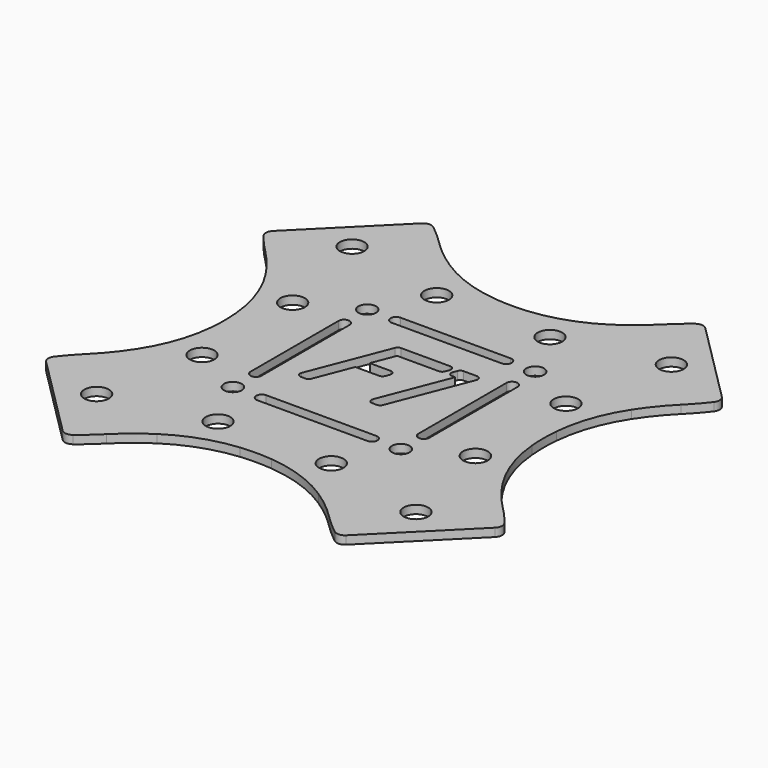
from build123d import *

# Parameters (mm, degrees)
F0_R     = 2.225
F0_R_2   = 1.6
F0_R_3   = 2.25
F1_DEPTH = 1.5


# Not quite as in the source:
# - ends of sketch curves that miss each other by under 0.0002 mm in the source are joined


with BuildPart() as f1:
    # F0 (on Top) → F1 (new body)
    with BuildSketch(Plane.XY):
        with BuildLine():
            Line((40.764131, 25.752812), (25.752812, 40.764131))
            ThreePointArc((25.752812, 40.764131), (24.7844707903, 41.2006273849), (23.7698381424, 40.8864068174))
            ThreePointArc((23.7698381424, 40.8864068174), (21.9550704325, 39.3793732762), (20.2364945752, 37.7635054248))
            ThreePointArc((20.2364945752, 37.7635054248), (17.5612326137, 35.3520830837), (14.6508446305, 33.2303795663))
            ThreePointArc((14.6508446305, 33.2303795663), (8.9914965544, 30.4470141229), (2.8299590067, 29.1013549294))
            ThreePointArc((2.8299590067, 29.1013549294), (0, 28.968262), (-2.8299590155, 29.1013548358))
            ThreePointArc((-2.8299590155, 29.1013548358), (-8.9914965544, 30.4470141229), (-14.6508445509, 33.2303796882))
            ThreePointArc((-14.6508445509, 33.2303796882), (-17.5612326137, 35.3520830837), (-20.2364941171, 37.7635058829))
            ThreePointArc((-20.2364941171, 37.7635058829), (-21.9550704325, 39.3793732762), (-23.7698383319, 40.8864065743))
            ThreePointArc((-23.7698383319, 40.8864065743), (-24.7844707903, 41.2006273849), (-25.7528121718, 40.7641311718))
            Line((-25.7528121718, 40.7641311718), (-40.764131, 25.752812))
            ThreePointArc((-40.764131, 25.752812), (-41.2006273849, 24.7844707903), (-40.8864068174, 23.7698381424))
            ThreePointArc((-40.8864068174, 23.7698381424), (-39.3793732762, 21.9550704325), (-37.7635054248, 20.2364945752))
            ThreePointArc((-37.7635054248, 20.2364945752), (-35.3520832558, 17.5612328258), (-33.2303798649, 14.6508450882))
            ThreePointArc((-33.2303798649, 14.6508450882), (-30.4470115556, 8.9914892045), (-29.1013534168, 2.8299429607))
            ThreePointArc((-29.1013534168, 2.8299429607), (-28.968262, 0), (-29.1013532045, -2.8299429807))
            ThreePointArc((-29.1013532045, -2.8299429807), (-30.4470115556, -8.9914892045), (-33.2303799868, -14.6508450086))
            ThreePointArc((-33.2303799868, -14.6508450086), (-35.3520832558, -17.5612328258), (-37.7635058829, -20.2364941171))
            ThreePointArc((-37.7635058829, -20.2364941171), (-39.3793732762, -21.9550704325), (-40.8864065743, -23.7698383319))
            ThreePointArc((-40.8864065743, -23.7698383319), (-41.2006273849, -24.7844707903), (-40.7641311718, -25.7528121718))
            Line((-40.7641311718, -25.7528121718), (-25.752812, -40.764131))
            ThreePointArc((-25.752812, -40.764131), (-24.7844707903, -41.2006273849), (-23.7698381424, -40.8864068174))
            ThreePointArc((-23.7698381424, -40.8864068174), (-21.9550704325, -39.3793732762), (-20.2364945752, -37.7635054248))
            ThreePointArc((-20.2364945752, -37.7635054248), (-17.5612326137, -35.3520830837), (-14.6508446305, -33.2303795663))
            ThreePointArc((-14.6508446305, -33.2303795663), (-8.9914965544, -30.4470141229), (-2.8299590067, -29.1013549294))
            ThreePointArc((-2.8299590067, -29.1013549294), (0, -28.968262), (2.8299590155, -29.1013548358))
            ThreePointArc((2.8299590155, -29.1013548358), (8.9914965544, -30.4470141229), (14.6508445509, -33.2303796882))
            ThreePointArc((14.6508445509, -33.2303796882), (17.5612326137, -35.3520830837), (20.2364941171, -37.7635058829))
            ThreePointArc((20.2364941171, -37.7635058829), (21.9550704325, -39.3793732762), (23.7698383319, -40.8864065743))
            ThreePointArc((23.7698383319, -40.8864065743), (24.7844707903, -41.2006273849), (25.7528121718, -40.7641311718))
            Line((25.7528121718, -40.7641311718), (40.764131, -25.752812))
            ThreePointArc((40.764131, -25.752812), (41.2006273849, -24.7844707903), (40.8864068174, -23.7698381424))
            ThreePointArc((40.8864068174, -23.7698381424), (39.3793732762, -21.9550704325), (37.7635054248, -20.2364945752))
            ThreePointArc((37.7635054248, -20.2364945752), (35.3520832558, -17.5612328258), (33.2303798649, -14.6508450882))
            ThreePointArc((33.2303798649, -14.6508450882), (30.4470115556, -8.9914892045), (29.1013534168, -2.8299429607))
            ThreePointArc((29.1013534168, -2.8299429607), (28.968262, 0), (29.1013532045, 2.8299429807))
            ThreePointArc((29.1013532045, 2.8299429807), (30.4470115556, 8.9914892045), (33.2303799868, 14.6508450086))
            ThreePointArc((33.2303799868, 14.6508450086), (35.3520832558, 17.5612328258), (37.7635058829, 20.2364941171))
            ThreePointArc((37.7635058829, 20.2364941171), (39.3793732762, 21.9550704325), (40.8864065743, 23.7698383319))
            ThreePointArc((40.8864065743, 23.7698383319), (41.2006273849, 24.7844707903), (40.764131, 25.752812))
        make_face()
        with Locations((-29, -29)):
            Circle(F0_R, mode=Mode.SUBTRACT)
        with Locations((-10.282726, -24.824696)):
            Circle(F0_R, mode=Mode.SUBTRACT)
        with Locations((-24.824696, -10.282726)):
            Circle(F0_R, mode=Mode.SUBTRACT)
        with Locations((-15.25, -15.25)):
            Circle(F0_R_2, mode=Mode.SUBTRACT)
        with Locations((10.282726, -24.824696)):
            Circle(F0_R, mode=Mode.SUBTRACT)
        with Locations((29, -29)):
            Circle(F0_R, mode=Mode.SUBTRACT)
        with BuildLine():
            Line((-10, -14.25), (10, -14.25))
            ThreePointArc((10, -14.25), (11, -15.25), (10, -16.25))
            Line((10, -16.25), (-10, -16.25))
            ThreePointArc((-10, -16.25), (-11, -15.25), (-10, -14.25))
        make_face(mode=Mode.SUBTRACT)
        with Locations((15.25, -15.25)):
            Circle(F0_R_2, mode=Mode.SUBTRACT)
        with Locations((24.824696, -10.282726)):
            Circle(F0_R_3, mode=Mode.SUBTRACT)
        with Locations((-24.824696, 10.282726)):
            Circle(F0_R, mode=Mode.SUBTRACT)
        with BuildLine():
            ThreePointArc((-16.25, 10), (-15.25, 11), (-14.25, 10))
            Line((-14.25, 10), (-14.25, -10))
            ThreePointArc((-14.25, -10), (-15.25, -11), (-16.25, -10))
            Line((-16.25, -10), (-16.25, 10))
        make_face(mode=Mode.SUBTRACT)
        with BuildLine():
            ThreePointArc((-0.4956958589, 0.885209945), (-0.771266673, 0.5382796173), (-1.194556, 0.407413))
            Line((-1.194556, 0.407413), (-5.541795, 0.407413))
            Line((-5.541795, 0.407413), (-8.150595, -6.290485))
            ThreePointArc((-8.150595, -6.290485), (-8.426165673, -6.6374153827), (-8.849455, -6.768282))
            Line((-8.849455, -6.768282), (-9.669691, -6.768282))
            ThreePointArc((-9.669691, -6.768282), (-10.2888243827, -6.441571327), (-10.3685511411, -5.746078945))
            Line((-10.3685511411, -5.746078945), (-4.809405, 8.526614))
            ThreePointArc((-4.809405, 8.526614), (-4.533834327, 8.8735443827), (-4.110545, 9.004411))
            Line((-4.110545, 9.004411), (4.809691, 9.004411))
            ThreePointArc((4.809691, 9.004411), (5.4288241198, 8.6777007117), (5.5085514793, 7.9822088133))
            Line((5.5085514793, 7.9822088133), (5.23237, 7.273132))
            ThreePointArc((5.23237, 7.273132), (4.9567984768, 6.9262017197), (4.533509, 6.795335))
            Line((4.533509, 6.795335), (-3.05373, 6.795335))
            Line((-3.05373, 6.795335), (-4.681371, 2.61649))
            Line((-4.681371, 2.61649), (-0.918374, 2.61649))
            ThreePointArc((-0.918374, 2.61649), (-0.2992406173, 2.289779327), (-0.2195138589, 1.594286945))
            Line((-0.2195138589, 1.594286945), (-0.4956958589, 0.885209945))
        make_face(mode=Mode.SUBTRACT)
        with Locations((-15.25, 15.25)):
            Circle(F0_R_2, mode=Mode.SUBTRACT)
        with Locations((-29, 29)):
            Circle(F0_R, mode=Mode.SUBTRACT)
        with Locations((-10.282726, 24.824696)):
            Circle(F0_R, mode=Mode.SUBTRACT)
        with BuildLine():
            ThreePointArc((3.290309, -6.768282), (2.6711756173, -6.441571327), (2.5914488589, -5.746078945))
            Line((2.5914488589, -5.746078945), (7.47627, 6.795335))
            Line((7.47627, 6.795335), (6.953273, 6.795335))
            ThreePointArc((6.953273, 6.795335), (6.3341396173, 7.122045673), (6.2544128589, 7.817538055))
            Line((6.2544128589, 7.817538055), (6.530595, 8.526614))
            ThreePointArc((6.530595, 8.526614), (6.806165673, 8.8735443827), (7.229455, 9.004411))
            Line((7.229455, 9.004411), (9.669691, 9.004411))
            ThreePointArc((9.669691, 9.004411), (10.2888241198, 8.6777007117), (10.3685514793, 7.9822088133))
            Line((10.3685514793, 7.9822088133), (4.809405, -6.290485))
            ThreePointArc((4.809405, -6.290485), (4.533834327, -6.6374153827), (4.110545, -6.768282))
            Line((4.110545, -6.768282), (3.290309, -6.768282))
        make_face(mode=Mode.SUBTRACT)
        with BuildLine():
            Line((14.25, -10), (14.25, 10))
            ThreePointArc((14.25, 10), (15.25, 11), (16.25, 10))
            Line((16.25, 10), (16.25, -10))
            ThreePointArc((16.25, -10), (15.25, -11), (14.25, -10))
        make_face(mode=Mode.SUBTRACT)
        with BuildLine():
            ThreePointArc((10, 16.25), (11, 15.25), (10, 14.25))
            Line((10, 14.25), (-10, 14.25))
            ThreePointArc((-10, 14.25), (-11, 15.25), (-10, 16.25))
            Line((-10, 16.25), (10, 16.25))
        make_face(mode=Mode.SUBTRACT)
        with Locations((15.25, 15.25)):
            Circle(F0_R_2, mode=Mode.SUBTRACT)
        with Locations((24.824696, 10.282726)):
            Circle(F0_R, mode=Mode.SUBTRACT)
        with Locations((10.282726, 24.824696)):
            Circle(F0_R, mode=Mode.SUBTRACT)
        with Locations((29, 29)):
            Circle(F0_R, mode=Mode.SUBTRACT)
    extrude(amount=F1_DEPTH)


solid = f1.part
